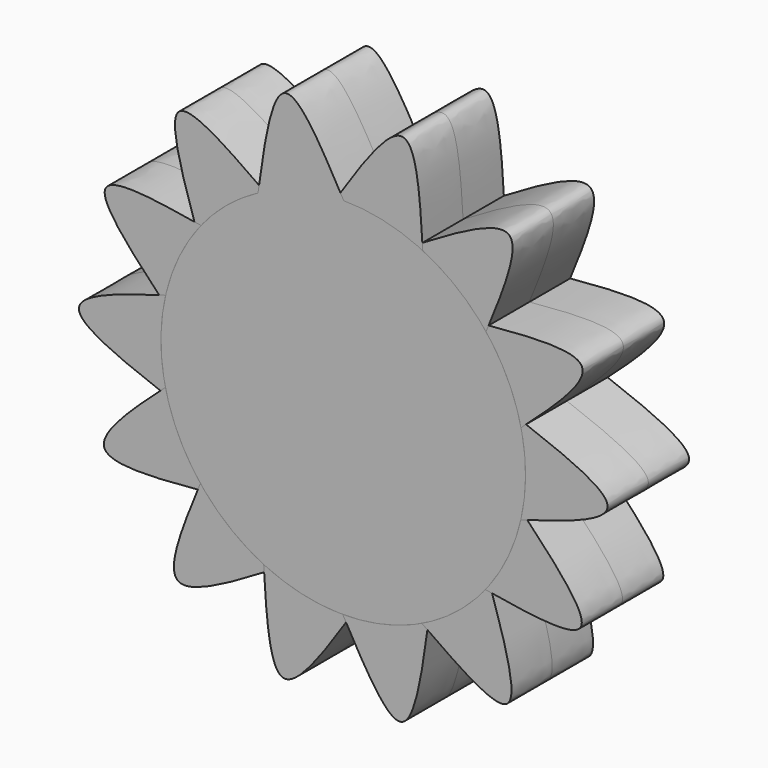
from build123d import *

# Parameters (mm, degrees)
F1_DEPTH = 12.7
F2_COUNT = 14
F4_D     = 38.1
F4_DEPTH = 12.7010001


with BuildPart() as f1:
    # F0 (on Front) → F1 (new body, symmetric)
    with BuildSketch(Plane.XZ):
        with BuildLine():
            ThreePointArc((-36.5605496231, 26.9586529359), (-14.1893429736, -43.1521181733), (45.4251335371, 0))
            ThreePointArc((45.4251335371, 0), (24.2229545258, 38.4277403825), (-19.5913503308, 40.9831886153))
            ThreePointArc((-19.5913503308, 40.9831886153), (-28.9383978023, 35.0144525803), (-36.5605496231, 26.9586529359))
        make_face()
        with BuildLine():
            ThreePointArc((-36.5605496231, 26.9586529359), (-28.9383978023, 35.0144525803), (-19.5913503308, 40.9831886153))
            add(Edge.make_bspline(
                [(-36.5605496231, 26.9586529359), (-40.1957905459, 38.2382410021), (-47.3220804985, 60.4589529461), (-28.7599156456, 47.4268803365), (-19.5913503308, 40.9831886153)],
                knots=[0, 0, 0, 0, 0.5067891827, 1, 1, 1, 1], degree=3))
        make_face()
    extrude(amount=F1_DEPTH, both=True)


with BuildPart() as f2_1:
    # F2: instance of F1
    add(f1.part.rotate(Axis((0, -12.7, 0), (0, -1, 0)), 1 * 360 / F2_COUNT))


with BuildPart() as f2_2:
    # F2: instance of F1
    add(f1.part.rotate(Axis((0, -12.7, 0), (0, -1, 0)), 2 * 360 / F2_COUNT))


with BuildPart() as f2_3:
    # F2: instance of F1
    add(f1.part.rotate(Axis((0, -12.7, 0), (0, -1, 0)), 3 * 360 / F2_COUNT))


with BuildPart() as f2_4:
    # F2: instance of F1
    add(f1.part.rotate(Axis((0, -12.7, 0), (0, -1, 0)), 4 * 360 / F2_COUNT))


with BuildPart() as f2_5:
    # F2: instance of F1
    add(f1.part.rotate(Axis((0, -12.7, 0), (0, -1, 0)), 5 * 360 / F2_COUNT))


with BuildPart() as f2_6:
    # F2: instance of F1
    add(f1.part.rotate(Axis((0, -12.7, 0), (0, -1, 0)), 6 * 360 / F2_COUNT))


with BuildPart() as f2_7:
    # F2: instance of F1
    add(f1.part.rotate(Axis((0, -12.7, 0), (0, -1, 0)), 7 * 360 / F2_COUNT))


with BuildPart() as f2_8:
    # F2: instance of F1
    add(f1.part.rotate(Axis((0, -12.7, 0), (0, -1, 0)), 8 * 360 / F2_COUNT))


with BuildPart() as f2_9:
    # F2: instance of F1
    add(f1.part.rotate(Axis((0, -12.7, 0), (0, -1, 0)), 9 * 360 / F2_COUNT))


with BuildPart() as f2_10:
    # F2: instance of F1
    add(f1.part.rotate(Axis((0, -12.7, 0), (0, -1, 0)), 10 * 360 / F2_COUNT))

    # F4 (through all, one way)
    with BuildSketch(Plane.XZ):
        with Locations((0, 0)):
            Circle(F4_D / 2)
    extrude(amount=-F4_DEPTH, mode=Mode.SUBTRACT)


with BuildPart() as f2_11:
    # F2: instance of F1
    add(f1.part.rotate(Axis((0, -12.7, 0), (0, -1, 0)), 11 * 360 / F2_COUNT))


with BuildPart() as f2_12:
    # F2: instance of F1
    add(f1.part.rotate(Axis((0, -12.7, 0), (0, -1, 0)), 12 * 360 / F2_COUNT))


with BuildPart() as f2_13:
    # F2: instance of F1
    add(f1.part.rotate(Axis((0, -12.7, 0), (0, -1, 0)), 13 * 360 / F2_COUNT))


solid = Compound([f1.part, f2_1.part, f2_2.part, f2_3.part, f2_4.part, f2_5.part, f2_6.part, f2_7.part, f2_8.part, f2_9.part, f2_10.part, f2_11.part, f2_12.part, f2_13.part])
